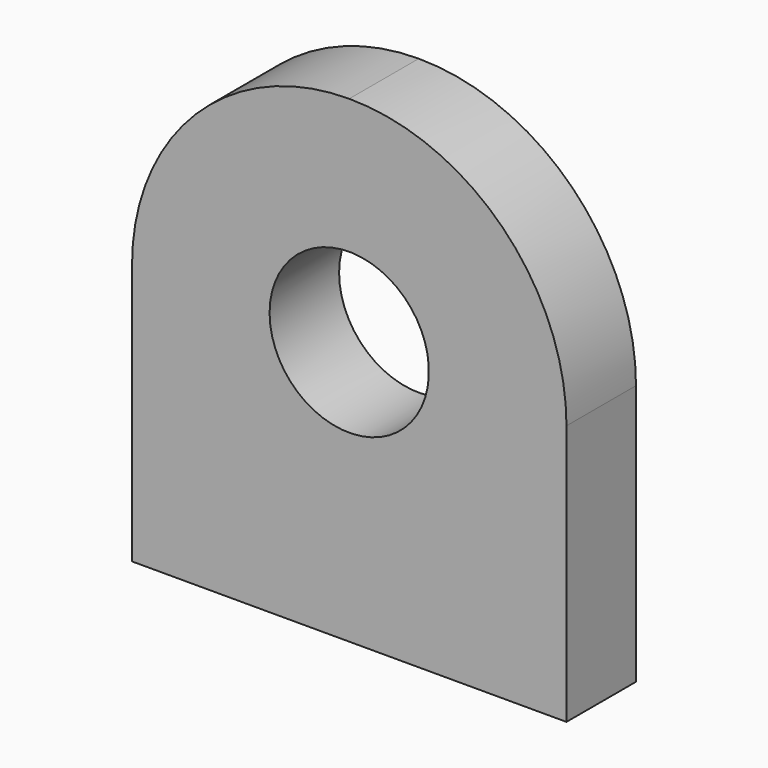
from build123d import *

# Parameters (mm, degrees)
F0_W     = 15
F0_H     = 3
F1_DEPTH = 16.5
F2_R     = 2.75
F3_DEPTH = 25
F4_R     = 7.49999


# Not quite as in the source:
# - a fillet or chamfer is up to 0.001 mm smaller than in the source, because OpenCascade refuses the exact size


with BuildPart() as f1:
    # F0 (on Top) → F1 (new body)
    with BuildSketch(Plane.XY):
        Rectangle(F0_W, F0_H)
    extrude(amount=F1_DEPTH)

    # F2 (on face) → F3 (cut)
    with BuildSketch(Plane(origin=(0, 1.5, 0), x_dir=(-1, 0, 0), z_dir=(0, 1, 0))):
        with Locations((0, 9.1)):
            Circle(F2_R)
    extrude(amount=-F3_DEPTH, mode=Mode.SUBTRACT)

    # F4 (radius 7.5 in the source; OpenCascade refuses exactly that, so slightly less here)
    f4_edges = [f1.edges().sort_by_distance(p)[0] for p in [
        (-7.5, 0, 16.5),
        (7.5, 0, 16.5),
    ]]
    fillet(f4_edges, radius=F4_R)


solid = f1.part
